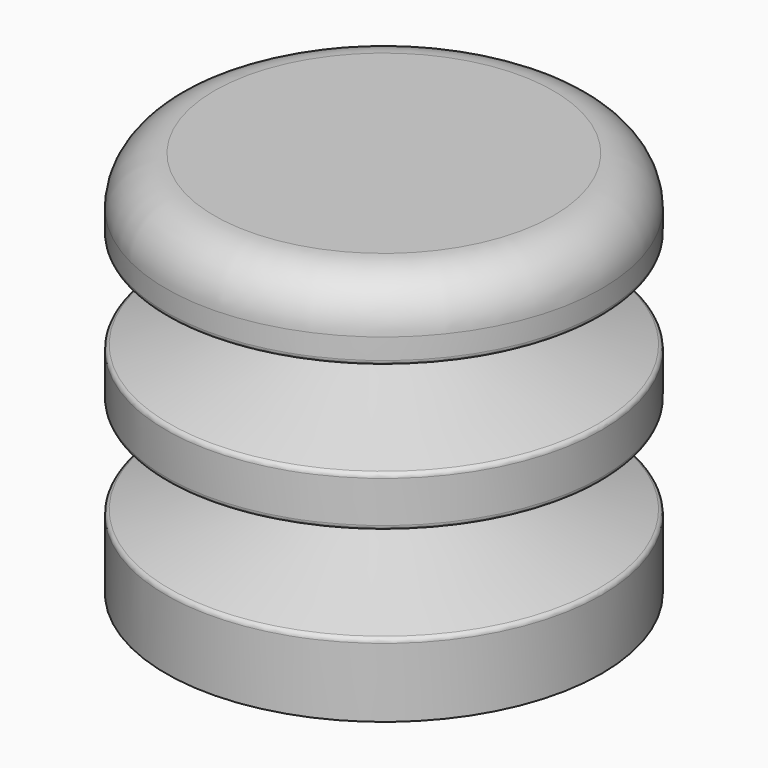
from build123d import *

# Parameters (mm, degrees)
F2_R     = 0.1
F5_DEPTH = 1
F6_DEPTH = 1
F7_R     = 1


with BuildPart() as f1:
    # F0 (on Front) → F1 (revolve)
    with BuildSketch(Plane.XZ):
        Polygon((0, 1.5), (0, 0), (4.5, 0), (4.5, 0.5), (2, 1.3333333333), (1.5, 1.5), align=None)
        Polygon((2, 1.5), (1.5, 1.5), (2, 1.3333333333), align=None)
    revolve(axis=Axis((0, 0, 0.75), (0, 0, 1)))

    # F2
    f2_edges = [f1.edges().sort_by_distance(p)[0] for p in [
        (-2, 0, 1.333333),
        (-4.5, 0, 0.5),
    ]]
    fillet(f2_edges, radius=F2_R)

    # F3: F1 across face


with BuildPart() as f1_1:
    add(f1.part)
    add(f1.part.mirror(Plane.XY.offset(1.5)))

    # F4: F1 across face


with BuildPart() as f1_2:
    add(f1_1.part)
    add(f1_1.part.mirror(Plane.XY.offset(3)))

    # F5 (add): a face of the model
    f5_faces = [f1_2.faces().sort_by_distance(p)[0] for p in [
        (0, 0, 6),
    ]]
    extrude(f5_faces, amount=F5_DEPTH)

    # F6 (add): a face of the model
    f6_faces = [f1_2.faces().sort_by_distance(p)[0] for p in [
        (0, 0, 0),
    ]]
    extrude(f6_faces, amount=F6_DEPTH)

    # F7
    f7_edges = [f1_2.edges().sort_by_distance(p)[0] for p in [
        (-4.5, 0, 7),
    ]]
    fillet(f7_edges, radius=F7_R)


solid = f1_2.part
